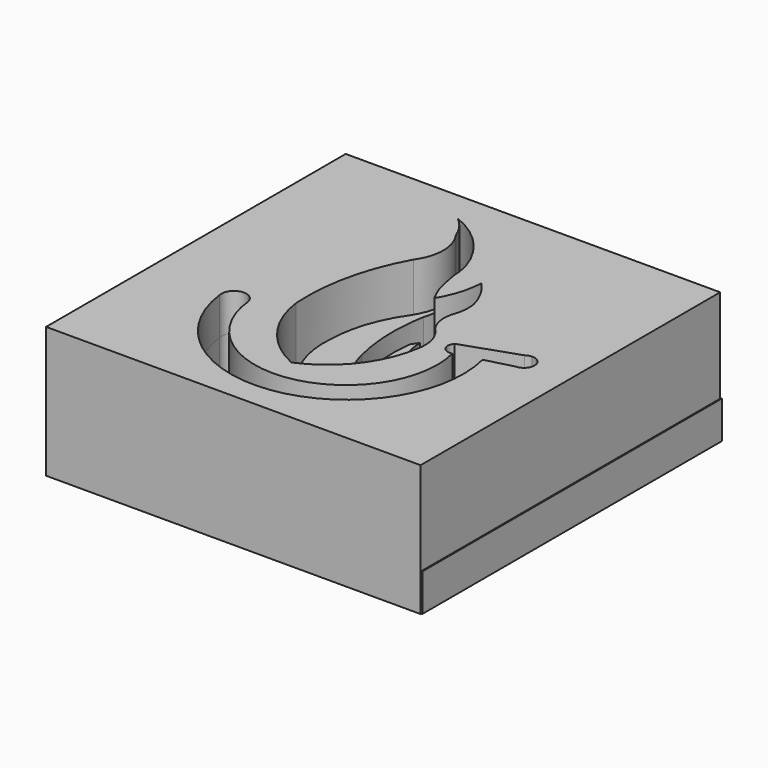
from build123d import *
from build123d import SkipClean  # not in build123d's __all__

# Parameters (mm, degrees)
F0_W      = 25.4
F0_H      = 25.4
F1_DEPTH  = 3.81
F3_DEPTH  = 6.35
F4_W      = 25.4
F4_H      = 25.4
F1_FACE_W = 25.4
F1_FACE_H = 25.4
F5_DEPTH  = 2.54
F7_DEPTH  = 3.81
F5_FACE_W = 25.4
F5_FACE_H = 25.4
F8_DEPTH  = 2.54
F9_DEPTH  = 6.35
F10_DEPTH = 5.08


# Not quite as in the source:
# - a feature names something its author has since deleted; it is built from what else it names


with BuildPart() as f1:
    # F0 (on Top) → F1 (new body)
    with BuildSketch(Plane.XY):
        Rectangle(F0_W, F0_H)
        with BuildLine():
            ThreePointArc((-2.3220747757, 5.493318662), (-1.7452180631, 7.2779146179), (-2.3220747757, 9.0625105738))
            ThreePointArc((-2.3220747757, 9.0625105738), (-2.7746823601, 9.912386532), (-3.427619813, 10.62006969))
            ThreePointArc((-3.427619813, 10.62006969), (-1.1425772736, 9.0743071478), (0.2757107432, 6.7080315202))
            ThreePointArc((0.2757107432, 6.7080315202), (0.4204105595, 6.0532877613), (0.4851105891, 5.3858738471))
            ThreePointArc((0.4851105891, 5.3858738471), (0.6353827008, 4.5817890382), (0.8147705941, 3.7836950142))
            ThreePointArc((0.8147705941, 3.7836950142), (1.0381967432, 3.2437817697), (1.2981665786, 2.7204833459))
            ThreePointArc((1.2981665786, 2.7204833459), (1.922383445, 4.1038367613), (2.1830380429, 5.5989529938))
            ThreePointArc((2.1830380429, 5.5989529938), (2.9114948167, 4.6138465954), (3.372413034, 3.4786645464))
            ThreePointArc((3.372413034, 3.4786645464), (3.4051009388, 2.7541360468), (3.2676233133, 2.0420195197))
            ThreePointArc((3.2676233133, 2.0420195197), (3.1432548322, 0.9887032001), (3.5271933302, 0))
            ThreePointArc((3.5271933302, 0), (4.1724784116, -1.0519502273), (4.2296264741, -2.2847219888))
            ThreePointArc((4.2296264741, -2.2847219888), (2.8346650657, -5.5849174863), (0, -7.7762370929))
            ThreePointArc((0, -7.7762370929), (-2.7435493808, -5.5658105565), (-4.0658875369, -2.3001604713))
            ThreePointArc((-4.0658875369, -2.3001604713), (-3.7552495624, 1.7221644716), (-2.3220747757, 5.493318662))
        make_face(mode=Mode.SUBTRACT)
    extrude(amount=F1_DEPTH)

    # F2 (on face) → F3 (cut)
    with BuildSketch(Plane.XY.offset(3.81)):
        with BuildLine():
            ThreePointArc((-6.1483882188, -3.7645904891), (-7.1429274149, -3.0984661258), (-7.8090517782, -4.0930053219))
            ThreePointArc((-7.8090517782, -4.0930053219), (1.9937266905, -10.7603517397), (7.3875300738, -0.2031334023))
            ThreePointArc((7.3875300738, -0.2031334023), (6.5005634578, -0.4457360723), (5.8456538245, -1.0912275175))
            ThreePointArc((5.8456538245, -1.0912275175), (1.3588648275, -9.2035644572), (-6.1483882188, -3.7645904891))
        make_face()
    extrude(amount=-F3_DEPTH, mode=Mode.SUBTRACT)



with BuildPart() as f1b:
    # F0 (on Top) → F1, piece 2 (new body)
    with BuildSketch(Plane.XY):
        with BuildLine():
            ThreePointArc((1.2607348617, 0), (-0.1199112872, 1.7654494083), (-0.65563916, 3.941682633))
            ThreePointArc((-0.65563916, 3.941682633), (-0.8248612998, 3.7079174894), (-0.9848921893, 3.4677667255))
            ThreePointArc((-0.9848921893, 3.4677667255), (-1.0263163384, 1.2153133206), (-0.671251677, -1.009364496))
            ThreePointArc((-0.671251677, -1.009364496), (0.2551522442, -3.0470440914), (1.8780454732, -4.5886601027))
            ThreePointArc((1.8780454732, -4.5886601027), (2.8324677453, -1.7438067709), (1.8650756683, 1.0966623668))
            ThreePointArc((1.8650756683, 1.0966623668), (1.7272115994, 0.4577864308), (1.2607348617, 0))
        make_face()
        with BuildLine():
            ThreePointArc((-0.671251677, -1.009364496), (-1.0263163384, 1.2153133206), (-0.9848921893, 3.4677667255))
            ThreePointArc((-0.9848921893, 3.4677667255), (-2.0972329272, -1.4632517602), (0.1975684196, -5.9672646379))
            ThreePointArc((0.1975684196, -5.9672646379), (1.0982734454, -5.351669196), (1.8780454732, -4.5886601027))
            ThreePointArc((1.8780454732, -4.5886601027), (0.2551522442, -3.0470440914), (-0.671251677, -1.009364496))
        make_face()
        with BuildLine():
            ThreePointArc((0.1975684196, -5.9672646379), (-2.0972329272, -1.4632517602), (-0.9848921893, 3.4677667255))
            ThreePointArc((-0.9848921893, 3.4677667255), (-0.9205654294, 3.97292477), (-0.8361481014, 4.4751162641))
            ThreePointArc((-0.8361481014, 4.4751162641), (-0.6366469014, 5.7604618421), (-0.8311524871, 7.0465728641))
            ThreePointArc((-0.8311524871, 7.0465728641), (-0.9366764425, 5.531166985), (-1.5578314768, 4.1448925869))
            ThreePointArc((-1.5578314768, 4.1448925869), (-2.6769387693, 1.8887344687), (-3.0985642225, -0.5941836862))
            ThreePointArc((-3.0985642225, -0.5941836862), (-2.5441879685, -3.7912333048), (-0.4829827521, -6.2972046435))
            ThreePointArc((-0.4829827521, -6.2972046435), (-0.1377056519, -6.1425510207), (0.1975684196, -5.9672646379))
        make_face()
    extrude(amount=F1_DEPTH)


with BuildPart() as f1_1:
    add(f1.part, clean=False)

    with SkipClean():  # cleaning this boolean's faces spoils the solid; the shape is the same uncleaned
        add(f1b.part)  # F5 merges F1b
    # F4 (on Top) + F1_face (on face) → F5 (join)
    with BuildSketch(Plane.XY):
        with Locations((0.066815722, 0.0637920246)):
            Rectangle(F4_W, F4_H)
    with BuildSketch(Plane(origin=(0.026992419, 0.041114738, 3.81), x_dir=(1, 0, 0), z_dir=(0, 0, 1))):
        with Locations((-0.026992419, -0.041114738)):
            Rectangle(F1_FACE_W, F1_FACE_H)
        with BuildLine():
            ThreePointArc((-7.8360441972, -4.1341200599), (-7.1699198339, -3.1395808638), (-6.1753806378, -3.805705227))
            ThreePointArc((-6.1753806378, -3.805705227), (1.3318724085, -9.2446791952), (5.8186614055, -1.1323422554))
            ThreePointArc((5.8186614055, -1.1323422554), (6.4735710387, -0.4868508103), (7.3605376548, -0.2442481402))
            ThreePointArc((7.3605376548, -0.2442481402), (1.9667342715, -10.8014664776), (-7.8360441972, -4.1341200599))
        make_face(mode=Mode.SUBTRACT)
        with BuildLine():
            ThreePointArc((-0.026992419, -7.8173518309), (-2.7705417999, -5.6069252945), (-4.0928799559, -2.3412752093))
            ThreePointArc((-4.0928799559, -2.3412752093), (-3.7822419814, 1.6810497336), (-2.3490671947, 5.4522039241))
            ThreePointArc((-2.3490671947, 5.4522039241), (-1.7722104822, 7.23679988), (-2.3490671947, 9.0213958359))
            ThreePointArc((-2.3490671947, 9.0213958359), (-2.8016747791, 9.871271794), (-3.454612232, 10.5789549521))
            ThreePointArc((-3.454612232, 10.5789549521), (-1.1695696926, 9.0331924098), (0.2487183241, 6.6669167823))
            ThreePointArc((0.2487183241, 6.6669167823), (0.3934181404, 6.0121730233), (0.4581181701, 5.3447591091))
            ThreePointArc((0.4581181701, 5.3447591091), (0.6083902818, 4.5406743002), (0.787778175, 3.7425802762))
            ThreePointArc((0.787778175, 3.7425802762), (1.0112043242, 3.2026670317), (1.2711741596, 2.6793686079))
            ThreePointArc((1.2711741596, 2.6793686079), (1.895391026, 4.0627220233), (2.1560456238, 5.5578382558))
            ThreePointArc((2.1560456238, 5.5578382558), (2.8845023977, 4.5727318574), (3.345420615, 3.4375498084))
            ThreePointArc((3.345420615, 3.4375498084), (3.3781085198, 2.7130213089), (3.2406308943, 2.0009047817))
            ThreePointArc((3.2406308943, 2.0009047817), (3.1162624132, 0.9475884621), (3.5002009112, -0.041114738))
            ThreePointArc((3.5002009112, -0.041114738), (4.1454859925, -1.0930649653), (4.2026340551, -2.3258367268))
            ThreePointArc((4.2026340551, -2.3258367268), (2.8076726467, -5.6260322243), (-0.026992419, -7.8173518309))
        make_face(mode=Mode.SUBTRACT)
    with SkipClean():  # cleaning this boolean's faces spoils the solid; the shape is the same uncleaned
        extrude(amount=F5_DEPTH)

    # F6 (on face) → F7 (cut)
    with BuildSketch(Plane.XY.offset(6.35)):
        with BuildLine():
            Line((9.553141892, 0.7298990968), (9.5194935584, 0.7182694883))
            ThreePointArc((9.5194935584, 0.7182694883), (9.5363131156, 0.7188602509), (9.553141892, 0.7190572078))
            Line((9.553141892, 0.7190572078), (9.553141892, 0.7298990968))
        make_face()
        with BuildLine():
            Line((9.1360899218, 0.5857567091), (5.4154974922, -0.7001623479))
            ThreePointArc((5.4154974922, -0.7001623479), (5.3482937998, -1.3922249308), (5.9925724035, -1.6537053999))
            Line((5.9925724035, -1.6537053999), (6.0142811862, -1.6480350907))
            ThreePointArc((6.0142811862, -1.6480350907), (5.9365127083, -1.3676491107), (5.8456538245, -1.0912275175))
            ThreePointArc((5.8456538245, -1.0912275175), (6.5005634578, -0.4457360723), (7.3875300738, -0.2031334023))
            ThreePointArc((7.3875300738, -0.2031334023), (7.5642186753, -0.6991201958), (7.7074975952, -1.2057689028))
            Line((7.7074975952, -1.2057689028), (9.5718006466, -0.7188150798))
            ThreePointArc((9.5718006466, -0.7188150798), (10.2721385652, 0.0093301628), (9.553141892, 0.7190572078))
            ThreePointArc((9.553141892, 0.7190572078), (9.5363131156, 0.7188602509), (9.5194935584, 0.7182694883))
            ThreePointArc((9.5194935584, 0.7182694883), (9.3182534076, 0.6796106738), (9.1360899218, 0.5857567091))
        make_face()
    with SkipClean():  # cleaning this boolean's faces spoils the solid; the shape is the same uncleaned
        extrude(amount=-F7_DEPTH, mode=Mode.SUBTRACT)

    # F0 (on Top) + F5_face (on face) → F8 (join)
    with BuildSketch(Plane.XY):
        with BuildLine():
            ThreePointArc((1.2607348617, 0), (-0.1199112872, 1.7654494083), (-0.65563916, 3.941682633))
            ThreePointArc((-0.65563916, 3.941682633), (-0.8248612998, 3.7079174894), (-0.9848921893, 3.4677667255))
            ThreePointArc((-0.9848921893, 3.4677667255), (-1.0263163384, 1.2153133206), (-0.671251677, -1.009364496))
            ThreePointArc((-0.671251677, -1.009364496), (0.2551522442, -3.0470440914), (1.8780454732, -4.5886601027))
            ThreePointArc((1.8780454732, -4.5886601027), (2.8324677453, -1.7438067709), (1.8650756683, 1.0966623668))
            ThreePointArc((1.8650756683, 1.0966623668), (1.7272115994, 0.4577864308), (1.2607348617, 0))
        make_face()
    with BuildSketch(Plane(origin=(-0.0427124334, 0.6105090747, 6.35), x_dir=(1, 0, 0), z_dir=(0, 0, 1))):
        with Locations((0.0427124334, -0.6105090747)):
            Rectangle(F5_FACE_W, F5_FACE_H)
        with BuildLine():
            ThreePointArc((-6.1056757855, -4.3750995638), (1.1161658852, -9.8706825468), (6.0569936196, -2.2585441654))
            Line((6.0569936196, -2.2585441654), (6.0352848369, -2.2642144746))
            ThreePointArc((6.0352848369, -2.2642144746), (5.3910062331, -2.0027340055), (5.4582099255, -1.3106714226))
            Line((5.4582099255, -1.3106714226), (9.1788023552, -0.0247523655))
            ThreePointArc((9.1788023552, -0.0247523655), (9.3609658409, 0.0691015992), (9.5622059917, 0.1077604136))
            Line((9.5622059917, 0.1077604136), (9.5958543253, 0.1193900221))
            Line((9.5958543253, 0.1193900221), (9.5958543253, 0.1085481331))
            ThreePointArc((9.5958543253, 0.1085481331), (10.3148509986, -0.6011789119), (9.61451308, -1.3293241545))
            Line((9.61451308, -1.3293241545), (7.7502100286, -1.8162779775))
            ThreePointArc((7.7502100286, -1.8162779775), (1.5223004235, -11.4843648142), (-7.7663393448, -4.7035143966))
            ThreePointArc((-7.7663393448, -4.7035143966), (-7.1002149816, -3.7089752005), (-6.1056757855, -4.3750995638))
        make_face(mode=Mode.SUBTRACT)
        with BuildLine():
            ThreePointArc((2.2257504762, 4.9884439191), (2.9542072501, 4.0033375207), (3.4151254674, 2.8681554717))
            ThreePointArc((3.4151254674, 2.8681554717), (3.4478133722, 2.1436269722), (3.3103357467, 1.431510445))
            ThreePointArc((3.3103357467, 1.431510445), (3.1859672656, 0.3781941254), (3.5699057636, -0.6105090747))
            ThreePointArc((3.5699057636, -0.6105090747), (4.2151908449, -1.662459302), (4.2723389075, -2.8952310635))
            ThreePointArc((4.2723389075, -2.8952310635), (2.877377499, -6.195426561), (0.0427124334, -8.3867461676))
            ThreePointArc((0.0427124334, -8.3867461676), (-2.7008369475, -6.1763196312), (-4.0231751035, -2.910669546))
            ThreePointArc((-4.0231751035, -2.910669546), (-3.712537129, 1.1116553969), (-2.2793623423, 4.8828095874))
            ThreePointArc((-2.2793623423, 4.8828095874), (-1.7025056298, 6.6674055433), (-2.2793623423, 8.4520014992))
            ThreePointArc((-2.2793623423, 8.4520014992), (-2.7319699267, 9.3018774573), (-3.3849073797, 10.0095606154))
            ThreePointArc((-3.3849073797, 10.0095606154), (-1.0998648402, 8.4637980731), (0.3184231765, 6.0975224456))
            ThreePointArc((0.3184231765, 6.0975224456), (0.4631229928, 5.4427786866), (0.5278230225, 4.7753647724))
            ThreePointArc((0.5278230225, 4.7753647724), (0.6780951342, 3.9712799635), (0.8574830274, 3.1731859395))
            ThreePointArc((0.8574830274, 3.1731859395), (1.0809091765, 2.633272695), (1.340879012, 2.1099742712))
            ThreePointArc((1.340879012, 2.1099742712), (1.9650958783, 3.4933276866), (2.2257504762, 4.9884439191))
        make_face(mode=Mode.SUBTRACT)
    extrude(amount=F8_DEPTH)

    # F0 (on Top) → F9 (join)
    with BuildSketch(Plane.XY):
        with BuildLine():
            ThreePointArc((0.1975684196, -5.9672646379), (-2.0972329272, -1.4632517602), (-0.9848921893, 3.4677667255))
            ThreePointArc((-0.9848921893, 3.4677667255), (-0.9205654294, 3.97292477), (-0.8361481014, 4.4751162641))
            ThreePointArc((-0.8361481014, 4.4751162641), (-0.6366469014, 5.7604618421), (-0.8311524871, 7.0465728641))
            ThreePointArc((-0.8311524871, 7.0465728641), (-0.9366764425, 5.531166985), (-1.5578314768, 4.1448925869))
            ThreePointArc((-1.5578314768, 4.1448925869), (-2.6769387693, 1.8887344687), (-3.0985642225, -0.5941836862))
            ThreePointArc((-3.0985642225, -0.5941836862), (-2.5441879685, -3.7912333048), (-0.4829827521, -6.2972046435))
            ThreePointArc((-0.4829827521, -6.2972046435), (-0.1377056519, -6.1425510207), (0.1975684196, -5.9672646379))
        make_face()
        with BuildLine():
            ThreePointArc((-0.671251677, -1.009364496), (-1.0263163384, 1.2153133206), (-0.9848921893, 3.4677667255))
            ThreePointArc((-0.9848921893, 3.4677667255), (-2.0972329272, -1.4632517602), (0.1975684196, -5.9672646379))
            ThreePointArc((0.1975684196, -5.9672646379), (1.0982734454, -5.351669196), (1.8780454732, -4.5886601027))
            ThreePointArc((1.8780454732, -4.5886601027), (0.2551522442, -3.0470440914), (-0.671251677, -1.009364496))
        make_face()
    extrude(amount=F9_DEPTH)

    # F0 (on Top) → F10 (join)
    with BuildSketch(Plane.XY):
        with BuildLine():
            ThreePointArc((1.2607348617, 0), (-0.1199112872, 1.7654494083), (-0.65563916, 3.941682633))
            ThreePointArc((-0.65563916, 3.941682633), (-0.8248612998, 3.7079174894), (-0.9848921893, 3.4677667255))
            ThreePointArc((-0.9848921893, 3.4677667255), (-1.0263163384, 1.2153133206), (-0.671251677, -1.009364496))
            ThreePointArc((-0.671251677, -1.009364496), (0.2551522442, -3.0470440914), (1.8780454732, -4.5886601027))
            ThreePointArc((1.8780454732, -4.5886601027), (2.8324677453, -1.7438067709), (1.8650756683, 1.0966623668))
            ThreePointArc((1.8650756683, 1.0966623668), (1.7272115994, 0.4577864308), (1.2607348617, 0))
        make_face()
    extrude(amount=F10_DEPTH)


solid = f1_1.part
